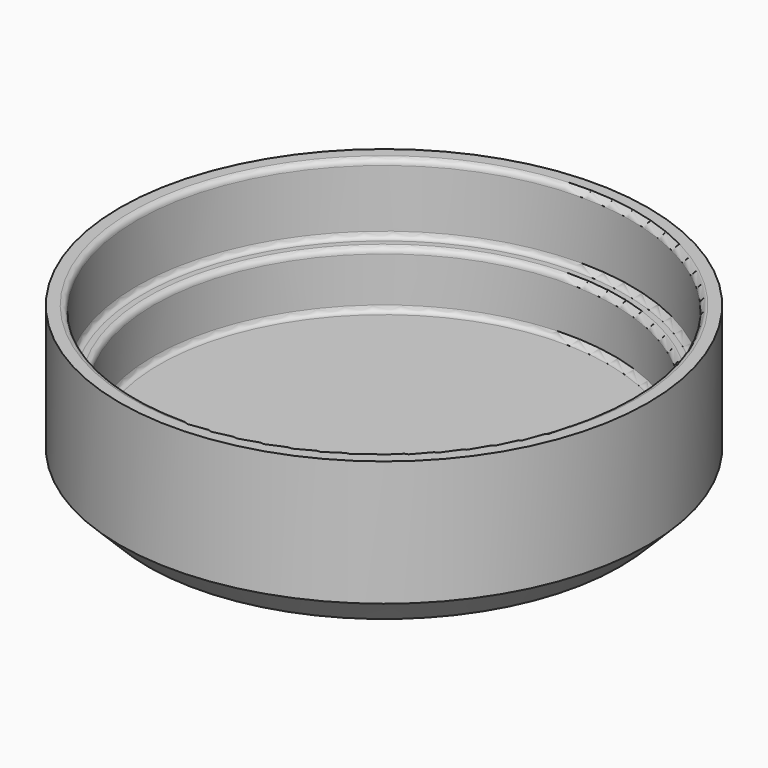
from build123d import *

# Parameters (mm, degrees)
F0_R     = 47
F0_R_2   = 44
F1_DEPTH = 22.3
F0_R_3   = 41
F2_DEPTH = 10
F3_DEPTH = 5
F4_R     = 1
F5_SIZE  = 4.99999


# Not quite as in the source:
# - a fillet or chamfer is up to 0.001 mm smaller than in the source, because OpenCascade refuses the exact size


with BuildPart() as f1:
    # F0 (on Top) → F1 (new body)
    with BuildSketch(Plane.XY):
        Circle(F0_R)
        Circle(F0_R_2, mode=Mode.SUBTRACT)
    extrude(amount=F1_DEPTH)

    # F0 (on Top) → F2 (join)
    with BuildSketch(Plane.XY):
        Circle(F0_R_2)
        Circle(F0_R_3, mode=Mode.SUBTRACT)
    extrude(amount=F2_DEPTH)

    # F0 (on Top) → F3 (join)
    with BuildSketch(Plane.XY):
        Circle(F0_R)
        Circle(F0_R_2, mode=Mode.SUBTRACT)
        Circle(F0_R_2)
        Circle(F0_R_3, mode=Mode.SUBTRACT)
        Circle(F0_R_3)
    extrude(amount=-F3_DEPTH)

    # F4
    f4_edges = [f1.edges().sort_by_distance(p)[0] for p in [
        (-44, 0, 22.3),
        (-44, 0, 10),
        (-41, 0, 10),
        (-41, 0, 0),
    ]]
    fillet(f4_edges, radius=F4_R)

    # F5 (size 5 in the source; OpenCascade refuses exactly that, so slightly less here)
    f5_edges = [f1.edges().sort_by_distance(p)[0] for p in [
        (-47, 0, -5),
    ]]
    chamfer(f5_edges, length=F5_SIZE)


solid = f1.part
